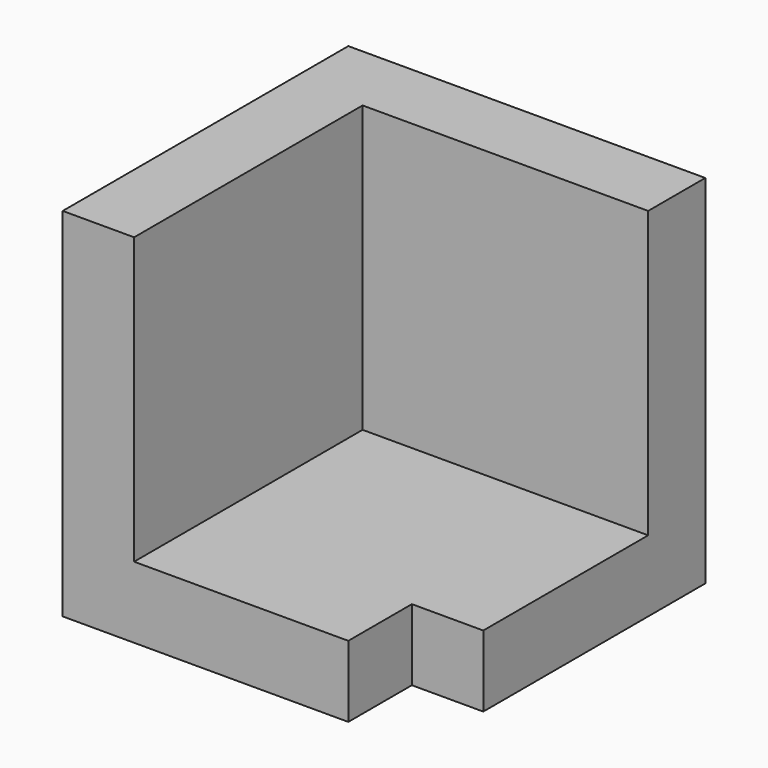
from build123d import *

# Parameters (mm, degrees)
F0_W     = 126.9999751441
F0_H     = 127
F1_DEPTH = 127
F2_W     = 25.4
F2_H     = 28.2670979543
F3_DEPTH = 127
F5_DEPTH = 101.6


# Not quite as in the source:
# - a feature names something its author has since deleted; it is built from what else it names


with BuildPart() as f1:
    # F0 (on Front) → F1 (new body)
    with BuildSketch(Plane.XZ):
        with Locations((63.4999875721, -63.5)):
            Rectangle(F0_W, F0_H)
    extrude(amount=F1_DEPTH)

    # F2 (on face) → F3 (cut)
    with BuildSketch(Plane.XY):
        with Locations((114.2999751441, -112.8664510228)):
            Rectangle(F2_W, F2_H)
    extrude(amount=-F3_DEPTH, mode=Mode.SUBTRACT)

    # F4 (on face) → F5 (cut)
    with BuildSketch(Plane.XY):
        Polygon((25.3999751441, -25.4), (25.3999751441, -127), (101.5999751441, -127), (101.5999751441, -98.7329020457), (126.9999751441, -98.7329020457), (126.9999751441, -25.4), align=None)
    extrude(amount=-F5_DEPTH, mode=Mode.SUBTRACT)


solid = f1.part
